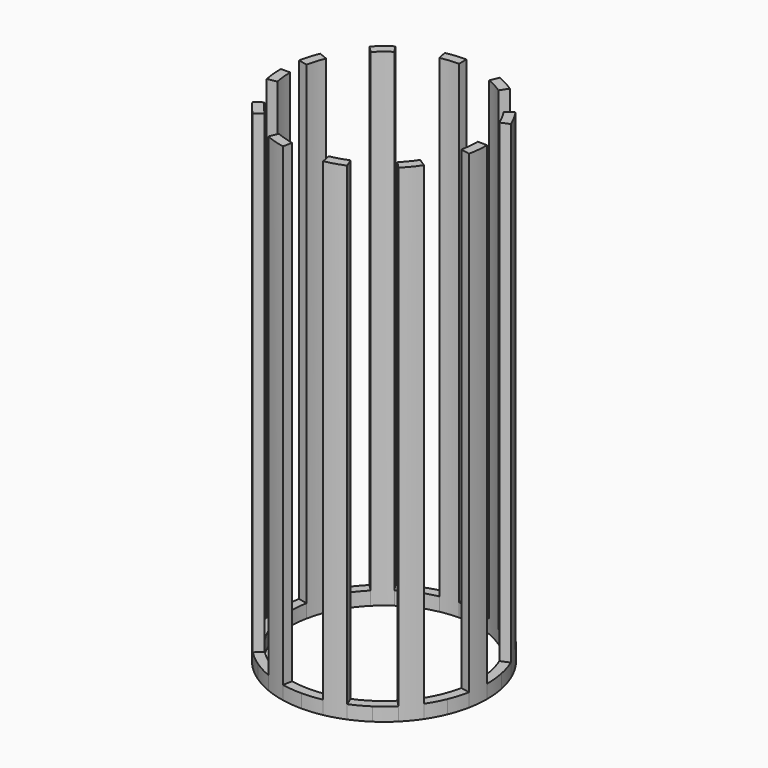
from build123d import *

# Parameters (mm, degrees)
F2_DEPTH = 3.6
F3_DEPTH = 130


with BuildPart() as f2:
    # F1 (on Top) → F2 (new body)
    with BuildSketch(Plane.XY):
        with BuildLine():
            Line((25, 0), (27.5, 0))
            ThreePointArc((27.5, 0), (27.3675799835, 2.6954713591), (26.9715952111, 5.3649838554))
            Line((26.9715952111, 5.3649838554), (24.5196320101, 4.8772580504))
            ThreePointArc((24.5196320101, 4.8772580504), (24.8796181668, 2.4504285082), (25, 0))
        make_face()
        with BuildLine():
            ThreePointArc((26.9715952111, -5.3649838554), (27.3675799835, -2.6954713591), (27.5, 0))
            Line((27.5, 0), (25, 0))
            ThreePointArc((25, 0), (24.8796181668, -2.4504285082), (24.5196320101, -4.8772580504))
            Line((24.5196320101, -4.8772580504), (26.9715952111, -5.3649838554))
        make_face()
        with BuildLine():
            Line((24.5196320101, 4.8772580504), (26.9715952111, 5.3649838554))
            ThreePointArc((26.9715952111, 5.3649838554), (26.3158592326, 7.9828286245), (25.4066871441, 10.52379439))
            Line((25.4066871441, 10.52379439), (23.0969883128, 9.5670858091))
            ThreePointArc((23.0969883128, 9.5670858091), (23.9235083933, 7.2571169314), (24.5196320101, 4.8772580504))
        make_face()
        with BuildLine():
            ThreePointArc((25.4066871441, -10.52379439), (26.3158592326, -7.9828286245), (26.9715952111, -5.3649838554))
            Line((26.9715952111, -5.3649838554), (24.5196320101, -4.8772580504))
            ThreePointArc((24.5196320101, -4.8772580504), (23.9235083933, -7.2571169314), (23.0969883128, -9.5670858091))
            Line((23.0969883128, -9.5670858091), (25.4066871441, -10.52379439))
        make_face()
        with BuildLine():
            Line((23.0969883128, 9.5670858091), (25.4066871441, 10.52379439))
            ThreePointArc((25.4066871441, 10.52379439), (24.2528347696, 12.9634102627), (22.8654143383, 15.278181408))
            Line((22.8654143383, 15.278181408), (20.7867403076, 13.8892558255))
            ThreePointArc((20.7867403076, 13.8892558255), (22.0480316087, 11.7849184207), (23.0969883128, 9.5670858091))
        make_face()
        with BuildLine():
            ThreePointArc((22.8654143383, -15.278181408), (24.2528347696, -12.9634102627), (25.4066871441, -10.52379439))
            Line((25.4066871441, -10.52379439), (23.0969883128, -9.5670858091))
            ThreePointArc((23.0969883128, -9.5670858091), (22.0480316087, -11.7849184207), (20.7867403076, -13.8892558255))
            Line((20.7867403076, -13.8892558255), (22.8654143383, -15.278181408))
        make_face()
        with BuildLine():
            Line((20.7867403076, 13.8892558255), (22.8654143383, 15.278181408))
            ThreePointArc((22.8654143383, 15.278181408), (21.2577874675, 17.4458153145), (19.4454364826, 19.4454364826))
            Line((19.4454364826, 19.4454364826), (17.6776695297, 17.6776695297))
            ThreePointArc((17.6776695297, 17.6776695297), (19.3252613341, 15.8598321041), (20.7867403076, 13.8892558255))
        make_face()
        with BuildLine():
            ThreePointArc((19.4454364826, -19.4454364826), (21.2577874675, -17.4458153145), (22.8654143383, -15.278181408))
            Line((22.8654143383, -15.278181408), (20.7867403076, -13.8892558255))
            ThreePointArc((20.7867403076, -13.8892558255), (19.3252613341, -15.8598321041), (17.6776695297, -17.6776695297))
            Line((17.6776695297, -17.6776695297), (19.4454364826, -19.4454364826))
        make_face()
        with BuildLine():
            Line((0, 27.5), (0, 25))
            ThreePointArc((0, 25), (2.4504285082, 24.8796181668), (4.8772580504, 24.5196320101))
            Line((4.8772580504, 24.5196320101), (5.3649838554, 26.9715952111))
            ThreePointArc((5.3649838554, 26.9715952111), (2.6954713591, 27.3675799835), (0, 27.5))
        make_face()
        with BuildLine():
            ThreePointArc((-4.8772580504, 24.5196320101), (-2.4504285082, 24.8796181668), (0, 25))
            Line((0, 25), (0, 27.5))
            ThreePointArc((0, 27.5), (-2.6954713591, 27.3675799835), (-5.3649838554, 26.9715952111))
            Line((-5.3649838554, 26.9715952111), (-4.8772580504, 24.5196320101))
        make_face()
        with BuildLine():
            Line((0, -27.5), (0, -25))
            ThreePointArc((0, -25), (-2.4504285082, -24.8796181668), (-4.8772580504, -24.5196320101))
            Line((-4.8772580504, -24.5196320101), (-5.3649838554, -26.9715952111))
            ThreePointArc((-5.3649838554, -26.9715952111), (-2.6954713591, -27.3675799835), (0, -27.5))
        make_face()
        with BuildLine():
            ThreePointArc((4.8772580504, -24.5196320101), (2.4504285082, -24.8796181668), (0, -25))
            Line((0, -25), (0, -27.5))
            ThreePointArc((0, -27.5), (2.6954713591, -27.3675799835), (5.3649838554, -26.9715952111))
            Line((5.3649838554, -26.9715952111), (4.8772580504, -24.5196320101))
        make_face()
        with BuildLine():
            Line((-27.5, 0), (-25, 0))
            ThreePointArc((-25, 0), (-24.8796181668, 2.4504285082), (-24.5196320101, 4.8772580504))
            Line((-24.5196320101, 4.8772580504), (-26.9715952111, 5.3649838554))
            ThreePointArc((-26.9715952111, 5.3649838554), (-27.3675799835, 2.6954713591), (-27.5, 0))
        make_face()
        with BuildLine():
            ThreePointArc((-24.5196320101, -4.8772580504), (-24.8796181668, -2.4504285082), (-25, 0))
            Line((-25, 0), (-27.5, 0))
            ThreePointArc((-27.5, 0), (-27.3675799835, -2.6954713591), (-26.9715952111, -5.3649838554))
            Line((-26.9715952111, -5.3649838554), (-24.5196320101, -4.8772580504))
        make_face()
        with BuildLine():
            Line((19.4454364826, -19.4454364826), (17.6776695297, -17.6776695297))
            ThreePointArc((17.6776695297, -17.6776695297), (15.8598321041, -19.3252613341), (13.8892558255, -20.7867403076))
            Line((13.8892558255, -20.7867403076), (15.278181408, -22.8654143383))
            ThreePointArc((15.278181408, -22.8654143383), (17.4458153145, -21.2577874675), (19.4454364826, -19.4454364826))
        make_face()
        with BuildLine():
            Line((10.52379439, -25.4066871441), (9.5670858091, -23.0969883128))
            ThreePointArc((9.5670858091, -23.0969883128), (7.2571169314, -23.9235083933), (4.8772580504, -24.5196320101))
            Line((4.8772580504, -24.5196320101), (5.3649838554, -26.9715952111))
            ThreePointArc((5.3649838554, -26.9715952111), (7.9828286245, -26.3158592326), (10.52379439, -25.4066871441))
        make_face()
        with BuildLine():
            ThreePointArc((13.8892558255, -20.7867403076), (11.7849184207, -22.0480316087), (9.5670858091, -23.0969883128))
            Line((9.5670858091, -23.0969883128), (10.52379439, -25.4066871441))
            ThreePointArc((10.52379439, -25.4066871441), (12.9634102627, -24.2528347696), (15.278181408, -22.8654143383))
            Line((15.278181408, -22.8654143383), (13.8892558255, -20.7867403076))
        make_face()
        with BuildLine():
            Line((-5.3649838554, -26.9715952111), (-4.8772580504, -24.5196320101))
            ThreePointArc((-4.8772580504, -24.5196320101), (-7.2571169314, -23.9235083933), (-9.5670858091, -23.0969883128))
            Line((-9.5670858091, -23.0969883128), (-10.52379439, -25.4066871441))
            ThreePointArc((-10.52379439, -25.4066871441), (-7.9828286245, -26.3158592326), (-5.3649838554, -26.9715952111))
        make_face()
        with BuildLine():
            Line((-10.52379439, -25.4066871441), (-9.5670858091, -23.0969883128))
            ThreePointArc((-9.5670858091, -23.0969883128), (-11.7849184207, -22.0480316087), (-13.8892558255, -20.7867403076))
            Line((-13.8892558255, -20.7867403076), (-15.278181408, -22.8654143383))
            ThreePointArc((-15.278181408, -22.8654143383), (-12.9634102627, -24.2528347696), (-10.52379439, -25.4066871441))
        make_face()
        with BuildLine():
            Line((-15.278181408, -22.8654143383), (-13.8892558255, -20.7867403076))
            ThreePointArc((-13.8892558255, -20.7867403076), (-15.8598321041, -19.3252613341), (-17.6776695297, -17.6776695297))
            Line((-17.6776695297, -17.6776695297), (-19.4454364826, -19.4454364826))
            ThreePointArc((-19.4454364826, -19.4454364826), (-17.4458153145, -21.2577874675), (-15.278181408, -22.8654143383))
        make_face()
        with BuildLine():
            Line((-19.4454364826, -19.4454364826), (-17.6776695297, -17.6776695297))
            ThreePointArc((-17.6776695297, -17.6776695297), (-19.3252613341, -15.8598321041), (-20.7867403076, -13.8892558255))
            Line((-20.7867403076, -13.8892558255), (-22.8654143383, -15.278181408))
            ThreePointArc((-22.8654143383, -15.278181408), (-21.2577874675, -17.4458153145), (-19.4454364826, -19.4454364826))
        make_face()
        with BuildLine():
            Line((-22.8654143383, -15.278181408), (-20.7867403076, -13.8892558255))
            ThreePointArc((-20.7867403076, -13.8892558255), (-22.0480316087, -11.7849184207), (-23.0969883128, -9.5670858091))
            Line((-23.0969883128, -9.5670858091), (-25.4066871441, -10.52379439))
            ThreePointArc((-25.4066871441, -10.52379439), (-24.2528347696, -12.9634102627), (-22.8654143383, -15.278181408))
        make_face()
        with BuildLine():
            Line((-25.4066871441, -10.52379439), (-23.0969883128, -9.5670858091))
            ThreePointArc((-23.0969883128, -9.5670858091), (-23.9235083933, -7.2571169314), (-24.5196320101, -4.8772580504))
            Line((-24.5196320101, -4.8772580504), (-26.9715952111, -5.3649838554))
            ThreePointArc((-26.9715952111, -5.3649838554), (-26.3158592326, -7.9828286245), (-25.4066871441, -10.52379439))
        make_face()
        with BuildLine():
            Line((-26.9715952111, 5.3649838554), (-24.5196320101, 4.8772580504))
            ThreePointArc((-24.5196320101, 4.8772580504), (-23.9235083933, 7.2571169314), (-23.0969883128, 9.5670858091))
            Line((-23.0969883128, 9.5670858091), (-25.4066871441, 10.52379439))
            ThreePointArc((-25.4066871441, 10.52379439), (-26.3158592326, 7.9828286245), (-26.9715952111, 5.3649838554))
        make_face()
        with BuildLine():
            Line((-25.4066871441, 10.52379439), (-23.0969883128, 9.5670858091))
            ThreePointArc((-23.0969883128, 9.5670858091), (-22.0480316087, 11.7849184207), (-20.7867403076, 13.8892558255))
            Line((-20.7867403076, 13.8892558255), (-22.8654143383, 15.278181408))
            ThreePointArc((-22.8654143383, 15.278181408), (-24.2528347696, 12.9634102627), (-25.4066871441, 10.52379439))
        make_face()
        with BuildLine():
            Line((-22.8654143383, 15.278181408), (-20.7867403076, 13.8892558255))
            ThreePointArc((-20.7867403076, 13.8892558255), (-19.3252613341, 15.8598321041), (-17.6776695297, 17.6776695297))
            Line((-17.6776695297, 17.6776695297), (-19.4454364826, 19.4454364826))
            ThreePointArc((-19.4454364826, 19.4454364826), (-21.2577874675, 17.4458153145), (-22.8654143383, 15.278181408))
        make_face()
        with BuildLine():
            Line((-19.4454364826, 19.4454364826), (-17.6776695297, 17.6776695297))
            ThreePointArc((-17.6776695297, 17.6776695297), (-15.8598321041, 19.3252613341), (-13.8892558255, 20.7867403076))
            Line((-13.8892558255, 20.7867403076), (-15.278181408, 22.8654143383))
            ThreePointArc((-15.278181408, 22.8654143383), (-17.4458153145, 21.2577874675), (-19.4454364826, 19.4454364826))
        make_face()
        with BuildLine():
            Line((-15.278181408, 22.8654143383), (-13.8892558255, 20.7867403076))
            ThreePointArc((-13.8892558255, 20.7867403076), (-11.7849184207, 22.0480316087), (-9.5670858091, 23.0969883128))
            Line((-9.5670858091, 23.0969883128), (-10.52379439, 25.4066871441))
            ThreePointArc((-10.52379439, 25.4066871441), (-12.9634102627, 24.2528347696), (-15.278181408, 22.8654143383))
        make_face()
        with BuildLine():
            Line((-10.52379439, 25.4066871441), (-9.5670858091, 23.0969883128))
            ThreePointArc((-9.5670858091, 23.0969883128), (-7.2571169314, 23.9235083933), (-4.8772580504, 24.5196320101))
            Line((-4.8772580504, 24.5196320101), (-5.3649838554, 26.9715952111))
            ThreePointArc((-5.3649838554, 26.9715952111), (-7.9828286245, 26.3158592326), (-10.52379439, 25.4066871441))
        make_face()
        with BuildLine():
            ThreePointArc((13.8892558255, 20.7867403076), (15.8598321041, 19.3252613341), (17.6776695297, 17.6776695297))
            Line((17.6776695297, 17.6776695297), (19.4454364826, 19.4454364826))
            ThreePointArc((19.4454364826, 19.4454364826), (17.4458153145, 21.2577874675), (15.278181408, 22.8654143383))
            Line((15.278181408, 22.8654143383), (13.8892558255, 20.7867403076))
        make_face()
        with BuildLine():
            ThreePointArc((9.5670858091, 23.0969883128), (11.7849184207, 22.0480316087), (13.8892558255, 20.7867403076))
            Line((13.8892558255, 20.7867403076), (15.278181408, 22.8654143383))
            ThreePointArc((15.278181408, 22.8654143383), (12.9634102627, 24.2528347696), (10.52379439, 25.4066871441))
            Line((10.52379439, 25.4066871441), (9.5670858091, 23.0969883128))
        make_face()
        with BuildLine():
            ThreePointArc((4.8772580504, 24.5196320101), (7.2571169314, 23.9235083933), (9.5670858091, 23.0969883128))
            Line((9.5670858091, 23.0969883128), (10.52379439, 25.4066871441))
            ThreePointArc((10.52379439, 25.4066871441), (7.9828286245, 26.3158592326), (5.3649838554, 26.9715952111))
            Line((5.3649838554, 26.9715952111), (4.8772580504, 24.5196320101))
        make_face()
    extrude(amount=F2_DEPTH)

    # F1 (on Top) → F3 (join)
    with BuildSketch(Plane.XY):
        with BuildLine():
            ThreePointArc((26.9715952111, -5.3649838554), (27.3675799835, -2.6954713591), (27.5, 0))
            Line((27.5, 0), (25, 0))
            ThreePointArc((25, 0), (24.8796181668, -2.4504285082), (24.5196320101, -4.8772580504))
            Line((24.5196320101, -4.8772580504), (26.9715952111, -5.3649838554))
        make_face()
        with BuildLine():
            ThreePointArc((19.4454364826, -19.4454364826), (21.2577874675, -17.4458153145), (22.8654143383, -15.278181408))
            Line((22.8654143383, -15.278181408), (20.7867403076, -13.8892558255))
            ThreePointArc((20.7867403076, -13.8892558255), (19.3252613341, -15.8598321041), (17.6776695297, -17.6776695297))
            Line((17.6776695297, -17.6776695297), (19.4454364826, -19.4454364826))
        make_face()
        with BuildLine():
            Line((10.52379439, -25.4066871441), (9.5670858091, -23.0969883128))
            ThreePointArc((9.5670858091, -23.0969883128), (7.2571169314, -23.9235083933), (4.8772580504, -24.5196320101))
            Line((4.8772580504, -24.5196320101), (5.3649838554, -26.9715952111))
            ThreePointArc((5.3649838554, -26.9715952111), (7.9828286245, -26.3158592326), (10.52379439, -25.4066871441))
        make_face()
        with BuildLine():
            Line((23.0969883128, 9.5670858091), (25.4066871441, 10.52379439))
            ThreePointArc((25.4066871441, 10.52379439), (24.2528347696, 12.9634102627), (22.8654143383, 15.278181408))
            Line((22.8654143383, 15.278181408), (20.7867403076, 13.8892558255))
            ThreePointArc((20.7867403076, 13.8892558255), (22.0480316087, 11.7849184207), (23.0969883128, 9.5670858091))
        make_face()
        with BuildLine():
            ThreePointArc((9.5670858091, 23.0969883128), (11.7849184207, 22.0480316087), (13.8892558255, 20.7867403076))
            Line((13.8892558255, 20.7867403076), (15.278181408, 22.8654143383))
            ThreePointArc((15.278181408, 22.8654143383), (12.9634102627, 24.2528347696), (10.52379439, 25.4066871441))
            Line((10.52379439, 25.4066871441), (9.5670858091, 23.0969883128))
        make_face()
        with BuildLine():
            ThreePointArc((-4.8772580504, 24.5196320101), (-2.4504285082, 24.8796181668), (0, 25))
            Line((0, 25), (0, 27.5))
            ThreePointArc((0, 27.5), (-2.6954713591, 27.3675799835), (-5.3649838554, 26.9715952111))
            Line((-5.3649838554, 26.9715952111), (-4.8772580504, 24.5196320101))
        make_face()
        with BuildLine():
            Line((-5.3649838554, -26.9715952111), (-4.8772580504, -24.5196320101))
            ThreePointArc((-4.8772580504, -24.5196320101), (-7.2571169314, -23.9235083933), (-9.5670858091, -23.0969883128))
            Line((-9.5670858091, -23.0969883128), (-10.52379439, -25.4066871441))
            ThreePointArc((-10.52379439, -25.4066871441), (-7.9828286245, -26.3158592326), (-5.3649838554, -26.9715952111))
        make_face()
        with BuildLine():
            Line((-19.4454364826, 19.4454364826), (-17.6776695297, 17.6776695297))
            ThreePointArc((-17.6776695297, 17.6776695297), (-15.8598321041, 19.3252613341), (-13.8892558255, 20.7867403076))
            Line((-13.8892558255, 20.7867403076), (-15.278181408, 22.8654143383))
            ThreePointArc((-15.278181408, 22.8654143383), (-17.4458153145, 21.2577874675), (-19.4454364826, 19.4454364826))
        make_face()
        with BuildLine():
            Line((-26.9715952111, 5.3649838554), (-24.5196320101, 4.8772580504))
            ThreePointArc((-24.5196320101, 4.8772580504), (-23.9235083933, 7.2571169314), (-23.0969883128, 9.5670858091))
            Line((-23.0969883128, 9.5670858091), (-25.4066871441, 10.52379439))
            ThreePointArc((-25.4066871441, 10.52379439), (-26.3158592326, 7.9828286245), (-26.9715952111, 5.3649838554))
        make_face()
        with BuildLine():
            Line((-19.4454364826, -19.4454364826), (-17.6776695297, -17.6776695297))
            ThreePointArc((-17.6776695297, -17.6776695297), (-19.3252613341, -15.8598321041), (-20.7867403076, -13.8892558255))
            Line((-20.7867403076, -13.8892558255), (-22.8654143383, -15.278181408))
            ThreePointArc((-22.8654143383, -15.278181408), (-21.2577874675, -17.4458153145), (-19.4454364826, -19.4454364826))
        make_face()
        with BuildLine():
            ThreePointArc((-24.5196320101, -4.8772580504), (-24.8796181668, -2.4504285082), (-25, 0))
            Line((-25, 0), (-27.5, 0))
            ThreePointArc((-27.5, 0), (-27.3675799835, -2.6954713591), (-26.9715952111, -5.3649838554))
            Line((-26.9715952111, -5.3649838554), (-24.5196320101, -4.8772580504))
        make_face()
    extrude(amount=F3_DEPTH)


solid = f2.part
